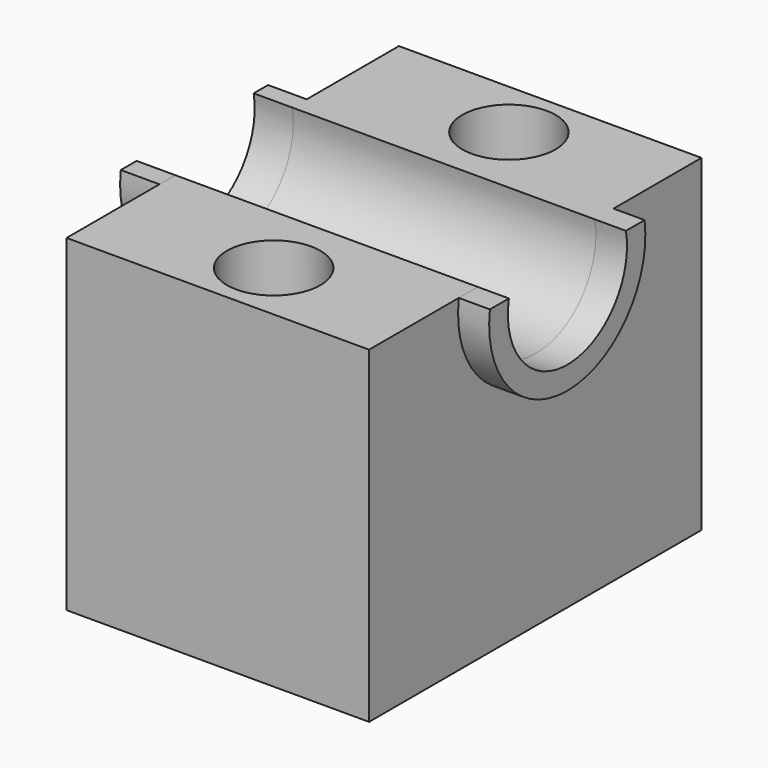
from build123d import *
from build123d import SkipClean  # not in build123d's __all__

# Parameters (mm, degrees)
F0_W     = 101.3660542667
F0_H     = 109.7881607711
F1_DEPTH = 69.596
F3_DEPTH = 101.3670542667
F5_DEPTH = 10.414
F7_DEPTH = 12.954
F8_R     = 15.6385789161
F9_DEPTH = 109.7891607711


# Not quite as in the source:
# - after a boolean that leaves OpenCascade's solid faulty, fix() repairs it


with BuildPart() as f1:
    # F0 (on Front) → F1 (new body, symmetric)
    with BuildSketch(Plane.XZ):
        with Locations((-2.2559221834, -7.3693413287)):
            Rectangle(F0_W, F0_H)
    extrude(amount=F1_DEPTH, both=True)

    # F2 (on face) → F3 (cut, through all)
    with BuildSketch(Plane.YZ.offset(48.42710495)):
        with BuildLine():
            Line((24.9655246735, 47.5247390568), (-24.0631587803, 47.5247390568))
            ThreePointArc((-24.0631587803, 47.5247390568), (0.4511829466, 18.0011880568), (24.9655246735, 47.5247390568))
        make_face()
    extrude(amount=-F3_DEPTH, mode=Mode.SUBTRACT)

    # F4 (on face) → F5 (join)
    with BuildSketch(Plane.YZ.offset(48.42710495)):
        with BuildLine():
            Line((-24.0631587803, 47.5247390568), (-32.028503716, 47.5247390568))
            ThreePointArc((-32.028503716, 47.5247390568), (0.372864306, 10.3342526114), (32.7742323279, 47.5247390568))
            Line((32.7742323279, 47.5247390568), (24.9655246735, 47.5247390568))
            ThreePointArc((24.9655246735, 47.5247390568), (0.4511829466, 18.0011880568), (-24.0631587803, 47.5247390568))
        make_face()
    with SkipClean():  # cleaning this boolean's faces spoils the solid; the shape is the same uncleaned
        extrude(amount=F5_DEPTH)

    # F6 (on face) → F7 (join)
    with BuildSketch(Plane(origin=(-52.9389493167, 0, 0), x_dir=(0, -1, 0), z_dir=(-1, 0, 0))):
        with BuildLine():
            Line((-24.9655246735, 47.5247390568), (-30.9813152999, 47.5247390568))
            ThreePointArc((-30.9813152999, 47.5247390568), (-0.1503955573, 12.1180891172), (30.6805241853, 47.5247390568))
            Line((30.6805241853, 47.5247390568), (24.0631587803, 47.5247390568))
            ThreePointArc((24.0631587803, 47.5247390568), (-0.4511829466, 18.0011880568), (-24.9655246735, 47.5247390568))
        make_face()
    extrude(amount=F7_DEPTH)

    add(f1.part.fix(), mode=Mode.REPLACE)

    # F8 (on face) → F9 (cut, through all)
    with BuildSketch(Plane.XY.offset(47.5247390568)):
        with Locations((0, 49.4834557176)):
            Circle(F8_R)
        with Locations((-2.8148e-06, -49.0286834538)):
            Circle(F8_R)
    extrude(amount=-F9_DEPTH, mode=Mode.SUBTRACT)


solid = f1.part
